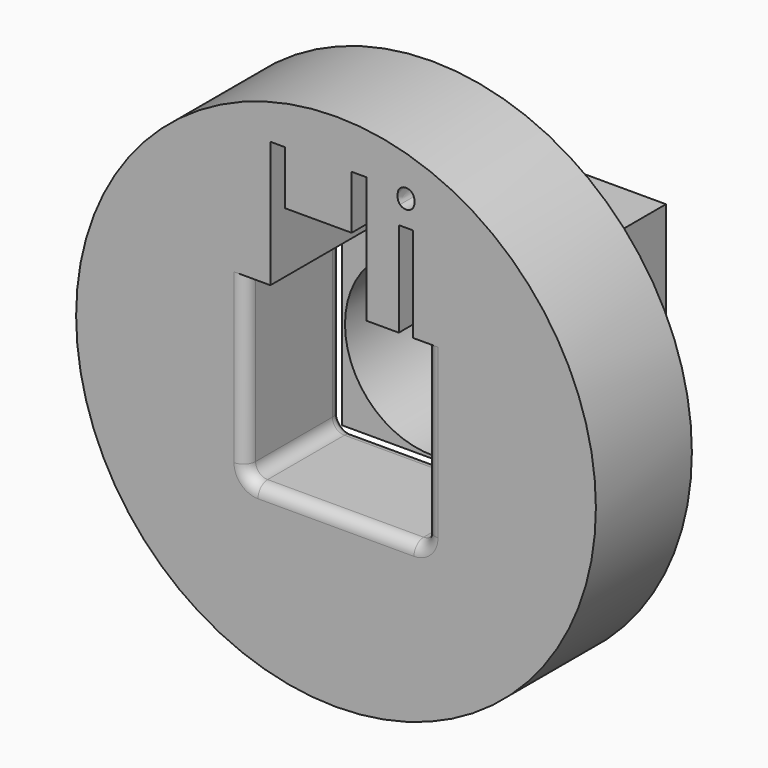
from build123d import *

# Parameters (mm, degrees)
F0_W     = 76.2
F0_H     = 76.2
F1_DEPTH = 76.2
F2_R     = 110.0290570582
F3_DEPTH = 50.8
F5_D     = 73.66
F6_R     = 5.08
F7_R     = 5.08


with BuildPart() as f1:
    # F0 (on Front) → F1 (new body)
    with BuildSketch(Plane.XZ):
        with Locations((-54.4605939882, 38.1)):
            Rectangle(F0_W, F0_H)
    extrude(amount=F1_DEPTH)

    # F5 (through all)
    with Locations(Plane.XZ.offset(76.2)):
        with Locations((-54.4605939882, 38.1)):
            Hole(F5_D / 2)


with BuildPart() as f3:
    # F2 (on face) → F3 (new body)
    with BuildSketch(Plane.XZ.offset(76.2)):
        with Locations((-54.4605939882, 38.1)):
            Circle(F2_R)
        Polygon((-41.6333082144, 129.6835716996), (-41.6333082144, 76.2), (-27.8790519774, 76.2), (-27.8790519774, 116.2921937122), (-21.8037677331, 116.2921937122), (-21.8037677331, 76.2), (-16.3605939882, 76.2), (-16.3605939882, 0), (-92.5605939882, 0), (-92.5605939882, 76.2), (-82.2405549261, 76.2), (-82.2405549261, 129.6835716996), (-76.024801682, 129.6835716996), (-76.024801682, 106.927593721), (-47.8490614585, 106.927593721), (-47.8490614585, 129.6835716996), align=None, mode=Mode.SUBTRACT)
        with BuildLine():
            add(Edge.make_bspline(
                [(-27.3698518528, 124.0999289549), (-28.3941049769, 125.1066234539), (-28.3941049769, 127.155129702)],
                knots=[0, 0, 0, 1, 1, 1], degree=2))
            add(Edge.make_bspline(
                [(-28.3941049769, 127.155129702), (-28.3941049769, 129.2387532), (-27.3698518528, 130.2103304491)],
                knots=[0, 0, 0, 1, 1, 1], degree=2))
            add(Edge.make_bspline(
                [(-27.3698518528, 130.2103304491), (-26.3455987288, 131.1819076982), (-24.8004397303, 131.1819076982)],
                knots=[0, 0, 0, 1, 1, 1], degree=2))
            add(Edge.make_bspline(
                [(-24.8004397303, 131.1819076982), (-23.3372209816, 131.1819076982), (-22.2778506076, 130.1927718241)],
                knots=[0, 0, 0, 1, 1, 1], degree=2))
            add(Edge.make_bspline(
                [(-22.2778506076, 130.1927718241), (-21.2184802336, 129.2036359501), (-21.2184802336, 127.155129702)],
                knots=[0, 0, 0, 1, 1, 1], degree=2))
            add(Edge.make_bspline(
                [(-21.2184802336, 127.155129702), (-21.2184802336, 125.1066234539), (-22.2778506076, 124.0999289549)],
                knots=[0, 0, 0, 1, 1, 1], degree=2))
            add(Edge.make_bspline(
                [(-22.2778506076, 124.0999289549), (-23.3372209816, 123.0932344558), (-24.8004397303, 123.0932344558)],
                knots=[0, 0, 0, 1, 1, 1], degree=2))
            add(Edge.make_bspline(
                [(-24.8004397303, 123.0932344558), (-26.3455987288, 123.0932344558), (-27.3698518528, 124.0999289549)],
                knots=[0, 0, 0, 1, 1, 1], degree=2))
        make_face(mode=Mode.SUBTRACT)
    extrude(amount=F3_DEPTH)

    # F6
    f6_edges = [f3.edges().sort_by_distance(p)[0] for p in [
        (55.568463, -101.6, 38.1),
        (-16.360594, -101.6, 0),
        (-16.360594, -127, 38.1),
        (-92.560594, -101.6, 0),
        (-54.460594, -127, 0),
        (-92.560594, -127, 38.1),
    ]]
    fillet(f6_edges, radius=F6_R)

    # F7
    f7_edges = [f3.edges().sort_by_distance(p)[0] for p in [
        (-54.460594, -76.2, 0),
        (-21.440594, -99.06, 0),
        (-87.480594, -99.06, 0),
        (-54.460594, -121.92, 0),
    ]]
    fillet(f7_edges, radius=F7_R)


solid = Compound([f1.part, f3.part])
